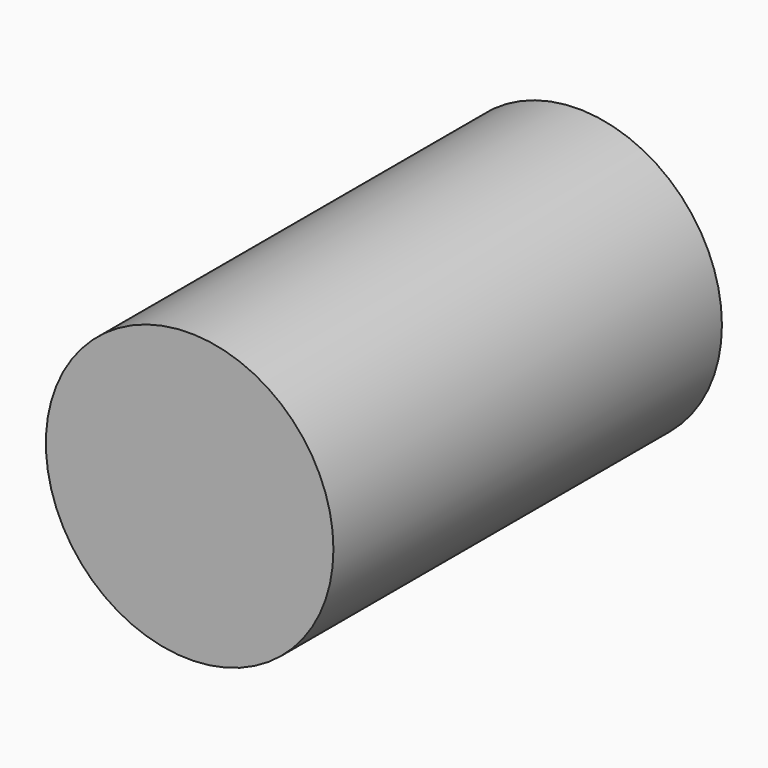
from build123d import *

# Parameters (mm, degrees)
F1_R     = 75.205752061
F2_DEPTH = 254


# Not quite as in the source:
# - the program builds the solid bodies; features that only make, move or delete a surface that nothing else refers to are left out


with BuildPart() as f2:
    # F1 (on face) → F2 (new body)
    with BuildSketch(Plane.XZ):
        Circle(F1_R)
    extrude(amount=F2_DEPTH)


solid = f2.part
